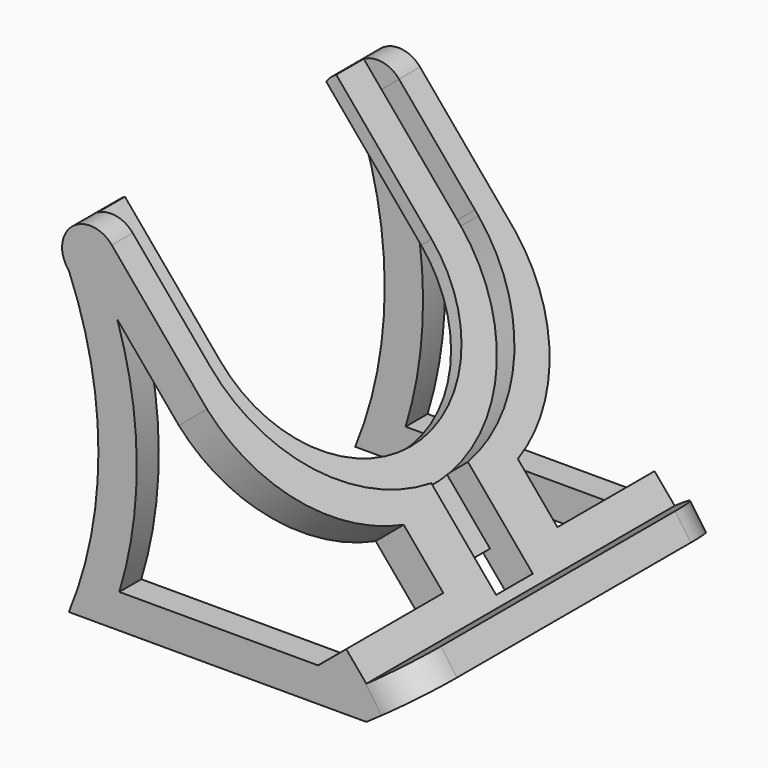
from build123d import *

# Parameters (mm, degrees)
F1_DEPTH  = 53.34
F2_W      = 9.5451793726
F2_H      = 32.1946403572
F3_DEPTH  = 6.35
F2_W_2    = 12.7
F2_H_2    = 9.3445232351
F4_DEPTH  = 7.62
F6_DEPTH  = 106.68
F8_W      = 91.44
F8_H      = 183.6228075896
F9_DEPTH  = 58.928
F10_DEPTH = 25.4
F11_DEPTH = 70.503420446
F12_R     = 12.8774151417
F13_DEPTH = 10.16


# Not quite as in the source:
# - a feature names something its author has since deleted; it is built from what else it names


with BuildPart() as f1:
    # F0 (on Front) → F1 (new body, symmetric)
    with BuildSketch(Plane.XZ):
        with BuildLine():
            ThreePointArc((-26.4580316219, 31.2050478526), (-18.2875299748, -10.3937397156), (-26.4580316219, -51.9925272838))
            Line((-26.4580316219, -51.9925272838), (55.8778569108, -51.9925272838))
            Line((55.8778569108, -51.9925272838), (70.650836429, -41.6293909539))
            Line((70.650836429, -41.6293909539), (66.2748063527, -35.3912212887))
            Line((66.2748063527, -35.3912212887), (55.8778569108, -42.6846047493))
            Line((55.8778569108, -42.6846047493), (-14.5902915946, 41.2960643955))
            ThreePointArc((-14.5902915946, 41.2960643955), (-25.6027276184, 42.2233043466), (-26.4580316219, 31.2050478526))
        make_face()
    extrude(amount=F1_DEPTH, both=True)

    # F2 (on face) → F3 (cut)
    with BuildSketch(Plane(origin=(11.772407622, 0, 9.8782228937), x_dir=(0, 1, 0), z_dir=(0.7660444431, 0, 0.6427876097))):
        with BuildLine():
            ThreePointArc((-36.5558206274, 35.6727858321), (-43.6495251277, 22.4172118106), (-46.101, 7.584101647))
            Line((-46.101, 7.584101647), (-36.5558206274, 7.584101647))
            Line((-36.5558206274, 7.584101647), (-36.5558206274, 35.6727858321))
        make_face()
        with BuildLine():
            Line((36.5558206274, 41.0130793115), (36.5558206274, 35.6727858321))
            ThreePointArc((36.5558206274, 35.6727858321), (43.5201114475, 22.7927209334), (46.0941562407, 8.3784324728))
            Line((46.0941562407, 8.3784324728), (46.0716254282, 41.0130793115))
            Line((46.0716254282, 41.0130793115), (36.5558206274, 41.0130793115))
        make_face()
        with BuildLine():
            Line((-36.5558206274, 41.0130793115), (-31.7459549124, 41.0130793115))
            ThreePointArc((-31.7459549124, 41.0130793115), (-17.0908294369, 50.4000536994), (0, 53.685101647))
            Line((0, 53.685101647), (0, 73.2077196687))
            Line((0, 73.2077196687), (-36.5558206274, 73.2077196687))
            Line((-36.5558206274, 73.2077196687), (-36.5558206274, 41.0130793115))
        make_face()
        with Locations((-41.3284103137, 57.1103994901)):
            Rectangle(F2_W, F2_H)
        Polygon((36.5558206274, 73.1040577223), (36.5558206274, 41.0130793115), (46.0716254282, 41.0130793115), (46.0494885484, 73.0771363708), align=None)
        with BuildLine():
            ThreePointArc((0, 53.685101647), (-17.0908294369, 50.4000536994), (-31.7459549124, 41.0130793115))
            Line((-31.7459549124, 41.0130793115), (-14.7929535268, 41.0130793115))
            ThreePointArc((-14.7929535268, 41.0130793115), (-7.5599044465, 43.3496698167), (0, 44.1399222744))
            Line((0, 44.1399222744), (0, 53.685101647))
        make_face()
        with BuildLine():
            ThreePointArc((31.7459549124, 41.0130793115), (17.0908294369, 50.4000536994), (0, 53.685101647))
            Line((0, 53.685101647), (0, 44.1399222744))
            ThreePointArc((0, 44.1399222744), (7.5599044465, 43.3496698167), (14.7929535268, 41.0130793115))
            Line((14.7929535268, 41.0130793115), (31.7459549124, 41.0130793115))
        make_face()
        with BuildLine():
            Line((-46.101, 41.0130793115), (-46.101, 7.584101647))
            ThreePointArc((-46.101, 7.584101647), (-43.6495251277, 22.4172118106), (-36.5558206274, 35.6727858321))
            Line((-36.5558206274, 35.6727858321), (-36.5558206274, 41.0130793115))
            Line((-36.5558206274, 41.0130793115), (-46.101, 41.0130793115))
        make_face()
        with BuildLine():
            Line((0, 73.2077196687), (0, 53.685101647))
            ThreePointArc((0, 53.685101647), (17.0908294369, 50.4000536994), (31.7459549124, 41.0130793115))
            Line((31.7459549124, 41.0130793115), (36.5558206274, 41.0130793115))
            Line((36.5558206274, 41.0130793115), (36.5558206274, 73.1040577223))
            Line((36.5558206274, 73.1040577223), (0, 73.2077196687))
        make_face()
        with BuildLine():
            Line((-36.5558206274, 41.0130793115), (-36.5558206274, 35.6727858321))
            ThreePointArc((-36.5558206274, 35.6727858321), (-34.2551137655, 38.4368062596), (-31.7459549124, 41.0130793115))
            Line((-31.7459549124, 41.0130793115), (-36.5558206274, 41.0130793115))
        make_face()
        with BuildLine():
            ThreePointArc((-31.7459549124, 41.0130793115), (-34.2551137655, 38.4368062596), (-36.5558206274, 35.6727858321))
            Line((-36.5558206274, 35.6727858321), (-36.5558206274, 7.584101647))
            ThreePointArc((-36.5558206274, 7.584101647), (-30.635735485, 27.5285177335), (-14.7929535268, 41.0130793115))
            Line((-14.7929535268, 41.0130793115), (-31.7459549124, 41.0130793115))
        make_face()
        with BuildLine():
            ThreePointArc((14.7929535268, 41.0130793115), (30.635735485, 27.5285177335), (36.5558206274, 7.584101647))
            Line((36.5558206274, 7.584101647), (36.5558206274, 35.6727858321))
            ThreePointArc((36.5558206274, 35.6727858321), (34.2551137655, 38.4368062596), (31.7459549124, 41.0130793115))
            Line((31.7459549124, 41.0130793115), (14.7929535268, 41.0130793115))
        make_face()
        with BuildLine():
            Line((-36.5558206274, 7.584101647), (-46.101, 7.584101647))
            ThreePointArc((-46.101, 7.584101647), (-34.7709904302, -22.686022659), (-6.35, -38.0774763043))
            ThreePointArc((-6.35, -38.0774763043), (0, -38.516898353), (6.35, -38.0774763043))
            ThreePointArc((6.35, -38.0774763043), (34.5300058488, -22.9606343493), (46.0952091038, 6.8534179416))
            Line((46.0952091038, 6.8534179416), (46.0941562407, 8.3784324728))
            ThreePointArc((46.0941562407, 8.3784324728), (43.5201114475, 22.7927209334), (36.5558206274, 35.6727858321))
            Line((36.5558206274, 35.6727858321), (36.5558206274, 7.584101647))
            ThreePointArc((36.5558206274, 7.584101647), (0, -28.9717189805), (-36.5558206274, 7.584101647))
        make_face()
        with BuildLine():
            Line((0, 7.584101647), (-36.5558206274, 7.584101647))
            ThreePointArc((-36.5558206274, 7.584101647), (0, -28.9717189805), (36.5558206274, 7.584101647))
            ThreePointArc((36.5558206274, 7.584101647), (30.635735485, 27.5285177335), (14.7929535268, 41.0130793115))
            Line((14.7929535268, 41.0130793115), (0, 41.0130793115))
            Line((0, 41.0130793115), (0, 7.584101647))
        make_face()
        with BuildLine():
            ThreePointArc((-14.7929535268, 41.0130793115), (-30.635735485, 27.5285177335), (-36.5558206274, 7.584101647))
            Line((-36.5558206274, 7.584101647), (0, 7.584101647))
            Line((0, 7.584101647), (0, 41.0130793115))
            Line((0, 41.0130793115), (-14.7929535268, 41.0130793115))
        make_face()
        with BuildLine():
            ThreePointArc((31.7459549124, 41.0130793115), (34.2551137655, 38.4368062596), (36.5558206274, 35.6727858321))
            Line((36.5558206274, 35.6727858321), (36.5558206274, 41.0130793115))
            Line((36.5558206274, 41.0130793115), (31.7459549124, 41.0130793115))
        make_face()
    extrude(amount=-F3_DEPTH, mode=Mode.SUBTRACT)

    # F2 (on face) → F4 (cut)
    with BuildSketch(Plane(origin=(11.772407622, 0, 9.8782228937), x_dir=(0, 1, 0), z_dir=(0.7660444431, 0, 0.6427876097))):
        with BuildLine():
            ThreePointArc((6.35, -38.0774763043), (0, -38.516898353), (-6.35, -38.0774763043))
            Line((-6.35, -38.0774763043), (-6.35, -56.6729530692))
            Line((-6.35, -56.6729530692), (6.35, -56.6729530692))
            Line((6.35, -56.6729530692), (6.35, -38.0774763043))
        make_face()
        with Locations((0, -61.3452146868)):
            Rectangle(F2_W_2, F2_H_2)
    extrude(amount=-F4_DEPTH, mode=Mode.SUBTRACT)

    # F5 (on face) → F6 (cut, through all)
    with BuildSketch(Plane.XZ.offset(53.34)):
        with BuildLine():
            Line((42.5035902841, -42.5519285295), (-13.0547319913, 23.6599016408))
            ThreePointArc((-13.0547319913, 23.6599016408), (-7.6819414216, -9.4041517757), (-12.5113723521, -42.5519285295))
            Line((-12.5113723521, -42.5519285295), (42.5035902841, -42.5519285295))
        make_face()
    extrude(amount=-F6_DEPTH, mode=Mode.SUBTRACT)

    # F8 (on face) → F9 (cut)
    with BuildSketch(Plane(origin=(-41.1275322828, 0, -34.5100971697), x_dir=(0, 1, 0), z_dir=(0.7660444431, 0, 0.6427876097))):
        with Locations((0, -8.2484856248)):
            Rectangle(F8_W, F8_H)
    extrude(amount=F9_DEPTH, mode=Mode.SUBTRACT)

    # F2 (on face) → F10 (cut)
    with BuildSketch(Plane(origin=(11.772407622, 0, 9.8782228937), x_dir=(0, 1, 0), z_dir=(0.7660444431, 0, 0.6427876097))):
        with BuildLine():
            ThreePointArc((-14.7929535268, 41.0130793115), (-30.635735485, 27.5285177335), (-36.5558206274, 7.584101647))
            Line((-36.5558206274, 7.584101647), (0, 7.584101647))
            Line((0, 7.584101647), (0, 41.0130793115))
            Line((0, 41.0130793115), (-14.7929535268, 41.0130793115))
        make_face()
        with BuildLine():
            Line((0, 7.584101647), (-36.5558206274, 7.584101647))
            ThreePointArc((-36.5558206274, 7.584101647), (0, -28.9717189805), (36.5558206274, 7.584101647))
            ThreePointArc((36.5558206274, 7.584101647), (30.635735485, 27.5285177335), (14.7929535268, 41.0130793115))
            Line((14.7929535268, 41.0130793115), (0, 41.0130793115))
            Line((0, 41.0130793115), (0, 7.584101647))
        make_face()
        with BuildLine():
            ThreePointArc((-31.7459549124, 41.0130793115), (-34.2551137655, 38.4368062596), (-36.5558206274, 35.6727858321))
            Line((-36.5558206274, 35.6727858321), (-36.5558206274, 7.584101647))
            ThreePointArc((-36.5558206274, 7.584101647), (-30.635735485, 27.5285177335), (-14.7929535268, 41.0130793115))
            Line((-14.7929535268, 41.0130793115), (-31.7459549124, 41.0130793115))
        make_face()
        with BuildLine():
            ThreePointArc((14.7929535268, 41.0130793115), (30.635735485, 27.5285177335), (36.5558206274, 7.584101647))
            Line((36.5558206274, 7.584101647), (36.5558206274, 35.6727858321))
            ThreePointArc((36.5558206274, 35.6727858321), (34.2551137655, 38.4368062596), (31.7459549124, 41.0130793115))
            Line((31.7459549124, 41.0130793115), (14.7929535268, 41.0130793115))
        make_face()
        with BuildLine():
            ThreePointArc((31.7459549124, 41.0130793115), (17.0908294369, 50.4000536994), (0, 53.685101647))
            Line((0, 53.685101647), (0, 44.1399222744))
            ThreePointArc((0, 44.1399222744), (7.5599044465, 43.3496698167), (14.7929535268, 41.0130793115))
            Line((14.7929535268, 41.0130793115), (31.7459549124, 41.0130793115))
        make_face()
        with BuildLine():
            ThreePointArc((0, 53.685101647), (-17.0908294369, 50.4000536994), (-31.7459549124, 41.0130793115))
            Line((-31.7459549124, 41.0130793115), (-14.7929535268, 41.0130793115))
            ThreePointArc((-14.7929535268, 41.0130793115), (-7.5599044465, 43.3496698167), (0, 44.1399222744))
            Line((0, 44.1399222744), (0, 53.685101647))
        make_face()
        with BuildLine():
            Line((-36.5558206274, 41.0130793115), (-31.7459549124, 41.0130793115))
            ThreePointArc((-31.7459549124, 41.0130793115), (-17.0908294369, 50.4000536994), (0, 53.685101647))
            Line((0, 53.685101647), (0, 73.2077196687))
            Line((0, 73.2077196687), (-36.5558206274, 73.2077196687))
            Line((-36.5558206274, 73.2077196687), (-36.5558206274, 41.0130793115))
        make_face()
        with BuildLine():
            Line((-36.5558206274, 41.0130793115), (-36.5558206274, 35.6727858321))
            ThreePointArc((-36.5558206274, 35.6727858321), (-34.2551137655, 38.4368062596), (-31.7459549124, 41.0130793115))
            Line((-31.7459549124, 41.0130793115), (-36.5558206274, 41.0130793115))
        make_face()
        with BuildLine():
            Line((0, 73.2077196687), (0, 53.685101647))
            ThreePointArc((0, 53.685101647), (17.0908294369, 50.4000536994), (31.7459549124, 41.0130793115))
            Line((31.7459549124, 41.0130793115), (36.5558206274, 41.0130793115))
            Line((36.5558206274, 41.0130793115), (36.5558206274, 73.1040577223))
            Line((36.5558206274, 73.1040577223), (0, 73.2077196687))
        make_face()
        with BuildLine():
            ThreePointArc((31.7459549124, 41.0130793115), (34.2551137655, 38.4368062596), (36.5558206274, 35.6727858321))
            Line((36.5558206274, 35.6727858321), (36.5558206274, 41.0130793115))
            Line((36.5558206274, 41.0130793115), (31.7459549124, 41.0130793115))
        make_face()
        with BuildLine():
            Line((0, 44.1399222744), (0, 41.0130793115))
            Line((0, 41.0130793115), (14.7929535268, 41.0130793115))
            ThreePointArc((14.7929535268, 41.0130793115), (7.5599044465, 43.3496698167), (0, 44.1399222744))
        make_face()
        with BuildLine():
            ThreePointArc((0, 44.1399222744), (-7.5599044465, 43.3496698167), (-14.7929535268, 41.0130793115))
            Line((-14.7929535268, 41.0130793115), (0, 41.0130793115))
            Line((0, 41.0130793115), (0, 44.1399222744))
        make_face()
    extrude(amount=-F10_DEPTH, mode=Mode.SUBTRACT)

    # F2 (on face) → F11 (cut, through all)
    with BuildSketch(Plane(origin=(11.772407622, 0, 9.8782228937), x_dir=(0, 1, 0), z_dir=(0.7660444431, 0, 0.6427876097))):
        with Locations((0, -61.3452146868)):
            Rectangle(F2_W_2, F2_H_2)
    extrude(amount=-F11_DEPTH, mode=Mode.SUBTRACT)

    # F12
    f12_edges = [f1.edges().sort_by_distance(p)[0] for p in [
        (68.462821, -53.34, -38.510306),
        (68.462821, 53.34, -38.510306),
    ]]
    fillet(f12_edges, radius=F12_R)

    # F2 (on face) → F13 (cut)
    with BuildSketch(Plane(origin=(11.772407622, 0, 9.8782228937), x_dir=(0, 1, 0), z_dir=(0.7660444431, 0, 0.6427876097))):
        with BuildLine():
            ThreePointArc((-19.7458926348, -42.8908065921), (-43.5565376092, -26.93877956), (-53.34, 0))
            Line((-53.34, 0), (-53.34, -59.9567629397))
            Line((-53.34, -59.9567629397), (-19.7458926348, -59.9567629397))
            Line((-19.7458926348, -59.9567629397), (-19.7458926348, -42.8908065921))
        make_face()
        with BuildLine():
            Line((53.34, -59.9567629397), (53.34, 0))
            ThreePointArc((53.34, 0), (43.5565376092, -26.93877956), (19.7458926348, -42.8908065921))
            Line((19.7458926348, -42.8908065921), (19.7458926348, -59.9567629397))
            Line((19.7458926348, -59.9567629397), (53.34, -59.9567629397))
        make_face()
    extrude(amount=-F13_DEPTH, mode=Mode.SUBTRACT)


solid = f1.part
